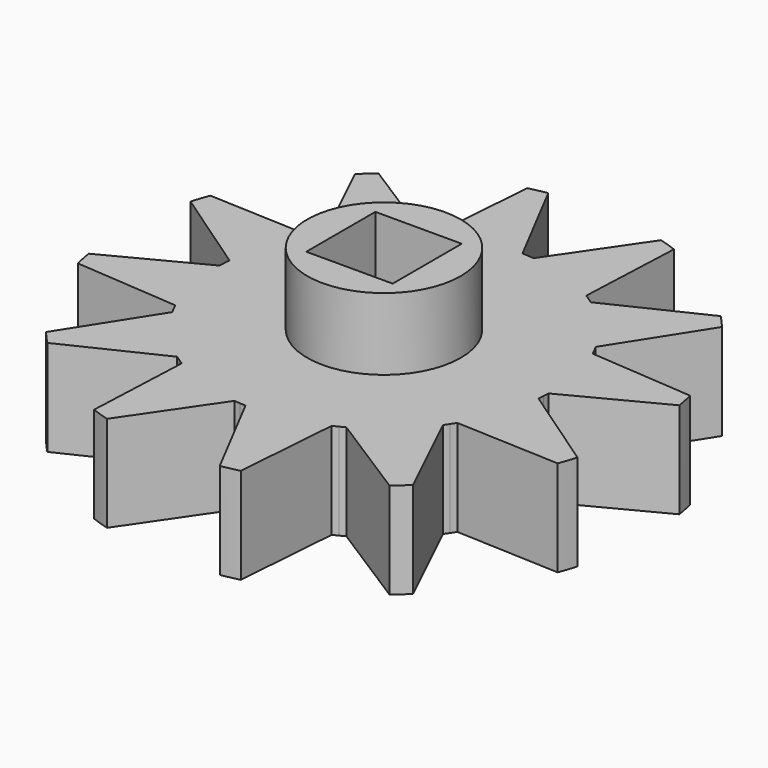
from build123d import *

# Parameters (mm, degrees)
F0_R            = 11
F1_DEPTH        = 4
F3_DEPTH        = 4.001
F3_COPIES_COUNT = 12
F5_R            = 3.2
F6_DEPTH        = 3
F7_W            = 3.6
F7_H            = 3.6
F8_DEPTH        = 7.001


# Not quite as in the source:
# - a pattern or mirror of a feature is missing from the dataset's text; its kind, count and spacing are read off the source's solid


with BuildPart() as f1:
    # F0 (on Top) → F1 (new body)
    with BuildSketch(Plane.XY):
        Circle(F0_R)
    extrude(amount=F1_DEPTH)

    # F2 (on face) → F3 (cut, through all)
    with BuildSketch(Plane.XY.offset(4)):
        with BuildLine():
            ThreePointArc((-3.3489182935, 6.1469298242), (-3.2411295194, 6.2044403002), (-3.1323534658, 6.2600608436))
            Line((-3.1323534658, 6.2600608436), (-4.922269732, 9.8372384685))
            ThreePointArc((-4.922269732, 9.8372384685), (-6.004235681, 9.2167865272), (-7.0090094429, 8.4778409179))
            Line((-7.0090094429, 8.4778409179), (-3.3489182935, 6.1469298242))
        make_face()
        with BuildLine():
            Line((-4.922269732, 9.8372384685), (-3.1323534658, 6.2600608436))
            ThreePointArc((-3.1323534658, 6.2600608436), (-3.022623267, 6.3137745118), (-2.9119723479, 6.3655649431))
            Line((-2.9119723479, 6.3655649431), (-2.5832151123, 10.6923804498))
            ThreePointArc((-2.5832151123, 10.6923804498), (-3.7770216625, 10.3312200326), (-4.922269732, 9.8372384685))
        make_face()
    f3 = extrude(amount=-F3_DEPTH, mode=Mode.SUBTRACT)

    # F3_copies: F3 ×12 about axis
    f3_copies_axis = Axis((0, 0, 0), (0, 0, 1))
    for i in range(1, F3_COPIES_COUNT):
        add(f3.rotate(f3_copies_axis, i * 360 / F3_COPIES_COUNT), mode=Mode.SUBTRACT)

    # F5 (on face) → F6 (join)
    with BuildSketch(Plane.XY.offset(4)):
        Circle(F5_R)
    extrude(amount=F6_DEPTH)

    # F7 (on face) → F8 (cut, through all)
    with BuildSketch(Plane.XY.offset(7)):
        Rectangle(F7_W, F7_H)
    extrude(amount=-F8_DEPTH, mode=Mode.SUBTRACT)


solid = f1.part
